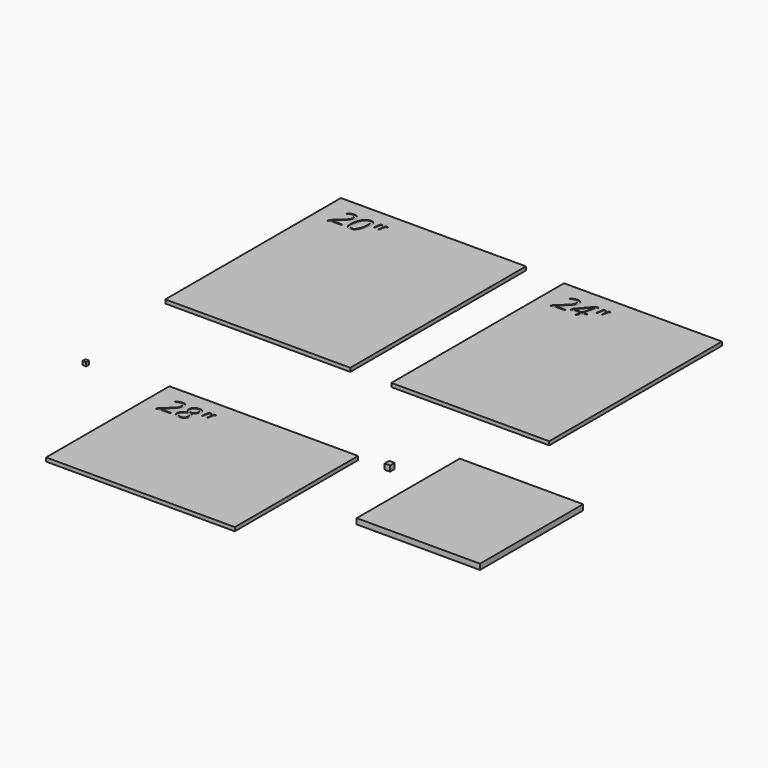
from build123d import *

# Parameters (mm, degrees)
F0_W          = 600
F0_H          = 712
F1_DEPTH      = 12
F2_W          = 512
F2_H          = 700
F3_DEPTH      = 12
F4_W          = 612
F4_H          = 500
F5_DEPTH      = 12
F6_W          = 12
F6_H          = 12
F7_DEPTH      = 12
F8_TEXT_SIZE  = 95.3232052428
F9_DEPTH      = 1.5
F10_TEXT_SIZE = 95.3232052428
F11_DEPTH     = 1.5
F12_TEXT_SIZE = 95.3232052428
F13_DEPTH     = 1.5
F14_W         = 400
F14_H         = 418
F15_DEPTH     = 18
F16_W         = 18
F16_H         = 18
F17_DEPTH     = 18


# Not quite as in the source:
# - Text() gives the source's letters only with a copy of the font that has no kerning and outlines rounded to 1/6400 em; it was checked with that copy


with BuildPart() as f1:
    # F0 (on Top) → F1 (new body)
    with BuildSketch(Plane.XY):
        with Locations((-300, 356)):
            Rectangle(F0_W, F0_H)
    extrude(amount=F1_DEPTH)

    # F8 (on face) → F9 (cut)
    with BuildSketch(Plane.XY.offset(12)):
        with Locations((-550, 593.3672922252)):
            Text('20"', F8_TEXT_SIZE, font='Open Sans', font_style=FontStyle.ITALIC, text_align=(TextAlign.LEFT, TextAlign.BOTTOM))
    extrude(amount=-F9_DEPTH, mode=Mode.SUBTRACT)


with BuildPart() as f3:
    # F2 (on Top) → F3 (new body)
    with BuildSketch(Plane.XY):
        with Locations((389.1459879875, 350)):
            Rectangle(F2_W, F2_H)
    extrude(amount=F3_DEPTH)

    # F10 (on face) → F11 (cut)
    with BuildSketch(Plane.XY.offset(12)):
        with Locations((183.1459879875, 581.3672922252)):
            Text('24"', F10_TEXT_SIZE, font='Open Sans', font_style=FontStyle.ITALIC, text_align=(TextAlign.LEFT, TextAlign.BOTTOM))
    extrude(amount=-F11_DEPTH, mode=Mode.SUBTRACT)


with BuildPart() as f5:
    # F4 (on Top) → F5 (new body)
    with BuildSketch(Plane.XY):
        with Locations((11.6966722012, -615.2527332306)):
            Rectangle(F4_W, F4_H)
    extrude(amount=F5_DEPTH)

    # F12 (on face) → F13 (cut)
    with BuildSketch(Plane.XY.offset(12)):
        with Locations((-244.3033277988, -483.8854410054)):
            Text('28"', F12_TEXT_SIZE, font='Open Sans', font_style=FontStyle.ITALIC, text_align=(TextAlign.LEFT, TextAlign.BOTTOM))
    extrude(amount=-F13_DEPTH, mode=Mode.SUBTRACT)


with BuildPart() as f7:
    # F6 (on Top) → F7 (new body)
    with BuildSketch(Plane.XY):
        with Locations((-547.0138964653, -388.2575454712)):
            Rectangle(F6_W, F6_H)
    extrude(amount=F7_DEPTH)


with BuildPart() as f15:
    # F14 (on Top) → F15 (new body)
    with BuildSketch(Plane.XY):
        with Locations((734.9998474121, -433.9998278618)):
            Rectangle(F14_W, F14_H)
    extrude(amount=F15_DEPTH)


with BuildPart() as f17:
    # F16 (on Top) → F17 (new body)
    with BuildSketch(Plane.XY):
        with Locations((411.649677515, -355.2520904541)):
            Rectangle(F16_W, F16_H)
    extrude(amount=F17_DEPTH)


solid = Compound([f1.part, f3.part, f5.part, f7.part, f15.part, f17.part])
